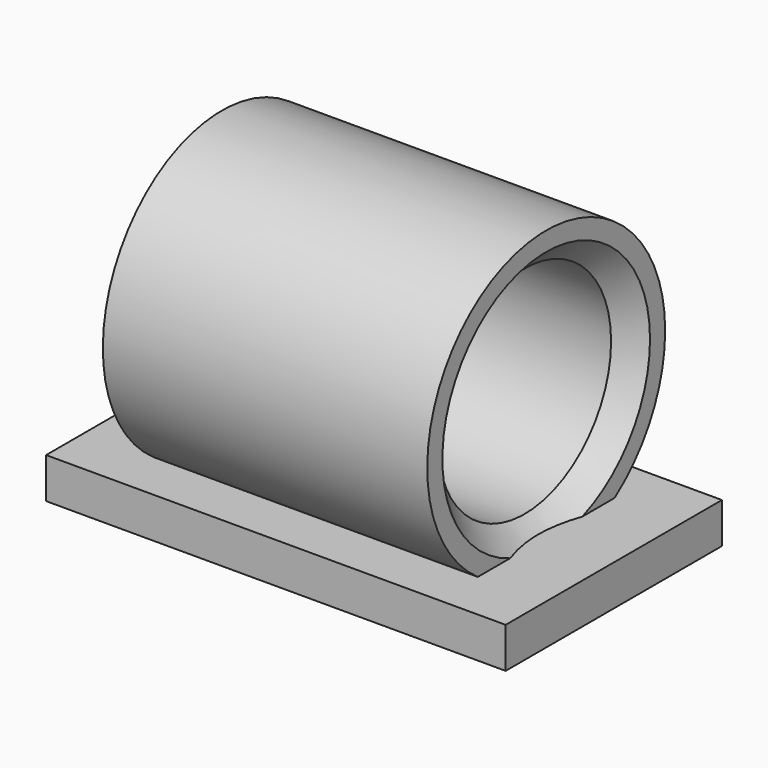
from build123d import *

# Parameters (mm, degrees)
F0_W     = 26.9875
F0_H     = 15.875
F1_DEPTH = 2.38125
F2_R     = 6.35
F3_DEPTH = 9.525


# Not quite as in the source:
# - a fillet or chamfer that OpenCascade refuses, or shapes differently, is made with other operations: its cross-section is extruded or revolved along the edge and cut away or added


with BuildPart() as f1:
    # F0 (on Top) → F1 (new body)
    with BuildSketch(Plane.XY):
        Rectangle(F0_W, F0_H)
    extrude(amount=F1_DEPTH)

    # F2 (on Right) → F3 (join, symmetric)
    with BuildSketch(Plane.YZ):
        with BuildLine():
            ThreePointArc((5.0201157855, 2.38125), (7.7481163038, 5.4999012055), (8.73125, 9.525))
            ThreePointArc((8.73125, 9.525), (-4.0250987945, 17.2731163038), (-5.0201157855, 2.38125))
            Line((-5.0201157855, 2.38125), (5.0201157855, 2.38125))
        make_face()
        with Locations((0, 9.525)):
            Circle(F2_R, mode=Mode.SUBTRACT)
    extrude(amount=F3_DEPTH, both=True)

    # F4: chamfer of 1.27 on 2 edges, made by hand


with BuildPart() as f4_tool2:
    # F4_s3 → F4_t4 (revolve)
    with BuildSketch(Plane.XY.offset(9.525)):
        Polygon((9.525, 7.62), (8.255, 6.35), (9.525, 6.35), align=None)
    revolve(axis=Axis((9.525, 0, 9.525), (1, 0, 0)))

    split(bisect_by=Plane.XY.offset(2.38125), keep=Keep.TOP)


with BuildPart() as f1_1:
    add(f1.part)

    # F4_t1: cut F4_tool2
    add(f4_tool2.part, mode=Mode.SUBTRACT)


with BuildPart() as f4_tool7:
    # F4_s8 → F4_t9 (revolve)
    with BuildSketch(Plane.XY.offset(9.525)):
        Polygon((-9.525, 7.62), (-8.255, 6.35), (-9.525, 6.35), align=None)
    revolve(axis=Axis((-9.525, 0, 9.525), (1, 0, 0)))

    split(bisect_by=Plane.XY.offset(2.38125), keep=Keep.TOP)


with BuildPart() as f1_2:
    add(f1_1.part)

    # F4_t6: cut F4_tool7
    add(f4_tool7.part, mode=Mode.SUBTRACT)


solid = f1_2.part
